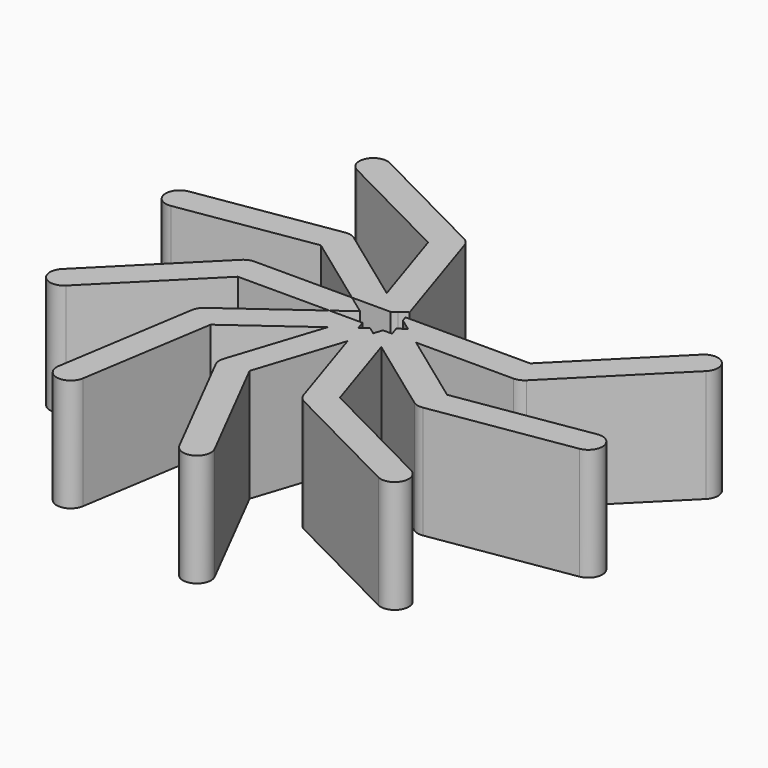
from build123d import *

# Parameters (mm, degrees)
F1_DEPTH = 25.4


# Not quite as in the source:
# - a feature names something its author has since deleted; it is built from what else it names


with BuildPart() as f1:
    # F0 (on Top) → F1 (new body)
    with BuildSketch(Plane.XY):
        with BuildLine():
            Line((9.7716452305, -3.175), (31.75, -3.175))
            ThreePointArc((31.75, -3.175), (32.9650198978, -2.9333175157), (33.9950640303, -2.2450640303))
            Line((33.9950640303, -2.2450640303), (56.4457043329, 20.2055762724))
            ThreePointArc((56.4457043329, 20.2055762724), (56.4457043329, 24.6957043329), (51.9555762724, 24.6957043329))
            Line((51.9555762724, 24.6957043329), (30.4348719395, 3.175))
            Line((30.4348719395, 3.175), (9.7716452305, 3.175))
            Line((9.7716452305, 3.175), (5.401632633, 0))
            Line((5.401632633, 0), (9.7716452305, -3.175))
        make_face()
        with BuildLine():
            Line((26.4885467967, -15.3205399243), (9.7716452305, -3.175))
            Line((9.7716452305, -3.175), (4.3700125975, -3.175))
            Line((4.3700125975, -3.175), (6.0392088785, -8.3122579143))
            Line((6.0392088785, -8.3122579143), (23.8200713954, -21.2308107174))
            ThreePointArc((23.8200713954, -21.2308107174), (24.9451005412, -21.7494562575), (26.1829689979, -21.7980922417))
            Line((26.1829689979, -21.7980922417), (57.5420738118, -16.8312979766))
            ThreePointArc((57.5420738118, -16.8312979766), (60.1813048667, -13.1987080688), (56.5487149588, -10.5594770139))
            Line((56.5487149588, -10.5594770139), (26.4885467967, -15.3205399243))
        make_face()
        Polygon((4.3700125975, -3.175), (9.7716452305, -3.175), (5.401632633, 0), (3.7324363521, -1.2127420857), align=None)
        Polygon((6.0392088785, -8.3122579143), (4.3700125975, -3.175), (2.3067725264, -3.175), (1.669196281, -5.1372579143), align=None)
        Polygon((2.7008163165, 1.9622579143), (5.401632633, 0), (9.7716452305, 3.175), (2.3067725264, 3.175), align=None)
        with BuildLine():
            Line((12.4244970902, -27.9641543235), (6.0392088785, -8.3122579143))
            Line((6.0392088785, -8.3122579143), (1.669196281, -5.1372579143))
            Line((1.669196281, -5.1372579143), (0, -10.2745158286))
            Line((0, -10.2745158286), (6.7916851322, -31.1771733495))
            ThreePointArc((6.7916851322, -31.1771733495), (7.3970006306, -32.2580419458), (8.3698697347, -33.0249901067))
            Line((8.3698697347, -33.0249901067), (36.6593268777, -47.4391884734))
            ThreePointArc((36.6593268777, -47.4391884734), (40.9296924287, -46.0516625958), (39.5421665511, -41.7812970448))
            Line((39.5421665511, -41.7812970448), (12.4244970902, -27.9641543235))
        make_face()
        Polygon((0, -10.2745158286), (1.669196281, -5.1372579143), (0, -3.9245158286), (-1.669196281, -5.1372579143), align=None)
        with BuildLine():
            Line((-6.3852882117, -29.9264122378), (0, -10.2745158286))
            Line((0, -10.2745158286), (-1.669196281, -5.1372579143))
            Line((-1.669196281, -5.1372579143), (-6.0392088785, -8.3122579143))
            Line((-6.0392088785, -8.3122579143), (-12.8308940106, -29.2149154352))
            ThreePointArc((-12.8308940106, -29.2149154352), (-12.976502106, -30.4451520213), (-12.6402352857, -31.637464229))
            Line((-12.6402352857, -31.637464229), (1.773963081, -59.926921372))
            ThreePointArc((1.773963081, -59.926921372), (6.044328632, -61.3144472496), (7.4318545096, -57.0440816987))
            Line((7.4318545096, -57.0440816987), (-6.3852882117, -29.9264122378))
        make_face()
        with BuildLine():
            Line((-6.0392088785, -8.3122579143), (-1.669196281, -5.1372579143))
            Line((-1.669196281, -5.1372579143), (-2.3067725264, -3.175))
            Line((-2.3067725264, -3.175), (-9.7716452305, -3.175))
            Line((-9.7716452305, -3.175), (-27.5525077474, -16.0935528031))
            ThreePointArc((-27.5525077474, -16.0935528031), (-28.3934220932, -17.0032488173), (-28.8222000528, -18.1655023338))
            Line((-28.8222000528, -18.1655023338), (-33.7889943178, -49.5246071477))
            ThreePointArc((-33.7889943178, -49.5246071477), (-31.1497632629, -53.1571970556), (-27.517173355, -50.5179660007))
            Line((-27.517173355, -50.5179660007), (-22.7561104446, -20.4577978386))
            Line((-22.7561104446, -20.4577978386), (-6.0392088785, -8.3122579143))
        make_face()
    extrude(amount=-F1_DEPTH)


with BuildPart() as f1b:
    # F0 (on Top) → F1, piece 2 (new body)
    with BuildSketch(Plane.XY):
        Polygon((0, 3.9245158286), (1.669196281, 5.1372579143), (0, 10.2745158286), (-1.669196281, 5.1372579143), align=None)
        Polygon((-1.0316200355, 3.175), (0, 3.9245158286), (-1.669196281, 5.1372579143), (-2.3067725264, 3.175), align=None)
        with BuildLine():
            Line((-1.669196281, 5.1372579143), (0, 10.2745158286))
            Line((0, 10.2745158286), (-6.7916851322, 31.1771733495))
            ThreePointArc((-6.7916851322, 31.1771733495), (-7.3970006306, 32.2580419458), (-8.3698697347, 33.0249901067))
            Line((-8.3698697347, 33.0249901067), (-36.6593268777, 47.4391884734))
            ThreePointArc((-36.6593268777, 47.4391884734), (-40.9296924287, 46.0516625958), (-39.5421665511, 41.7812970448))
            Line((-39.5421665511, 41.7812970448), (-12.4244970902, 27.9641543235))
            Line((-12.4244970902, 27.9641543235), (-6.0392088785, 8.3122579143))
            Line((-6.0392088785, 8.3122579143), (-1.669196281, 5.1372579143))
        make_face()
        Polygon((-2.3067725264, 3.175), (-1.669196281, 5.1372579143), (-6.0392088785, 8.3122579143), (-4.3700125975, 3.175), align=None)
        with BuildLine():
            Line((-4.3700125975, 3.175), (-6.0392088785, 8.3122579143))
            Line((-6.0392088785, 8.3122579143), (-23.8200713954, 21.2308107174))
            ThreePointArc((-23.8200713954, 21.2308107174), (-24.9451005412, 21.7494562575), (-26.1829689979, 21.7980922417))
            Line((-26.1829689979, 21.7980922417), (-57.5420738118, 16.8312979766))
            ThreePointArc((-57.5420738118, 16.8312979766), (-60.1813048667, 13.1987080688), (-56.5487149588, 10.5594770139))
            Line((-56.5487149588, 10.5594770139), (-26.4885467967, 15.3205399243))
            Line((-26.4885467967, 15.3205399243), (-9.7716452305, 3.175))
            Line((-9.7716452305, 3.175), (-4.3700125975, 3.175))
        make_face()
    extrude(amount=-F1_DEPTH)


with BuildPart() as f1c:
    # F0 (on Top) → F1, piece 3 (new body)
    with BuildSketch(Plane.XY):
        with BuildLine():
            Line((-30.4348719395, -3.175), (-9.7716452305, -3.175))
            Line((-9.7716452305, -3.175), (-5.401632633, 0))
            Line((-5.401632633, 0), (-9.7716452305, 3.175))
            Line((-9.7716452305, 3.175), (-31.75, 3.175))
            ThreePointArc((-31.75, 3.175), (-32.9650198978, 2.9333175157), (-33.9950640303, 2.2450640303))
            Line((-33.9950640303, 2.2450640303), (-56.4457043329, -20.2055762724))
            ThreePointArc((-56.4457043329, -20.2055762724), (-56.4457043329, -24.6957043329), (-51.9555762724, -24.6957043329))
            Line((-51.9555762724, -24.6957043329), (-30.4348719395, -3.175))
        make_face()
    extrude(amount=-F1_DEPTH)


solid = Compound([f1.part, f1b.part, f1c.part])
